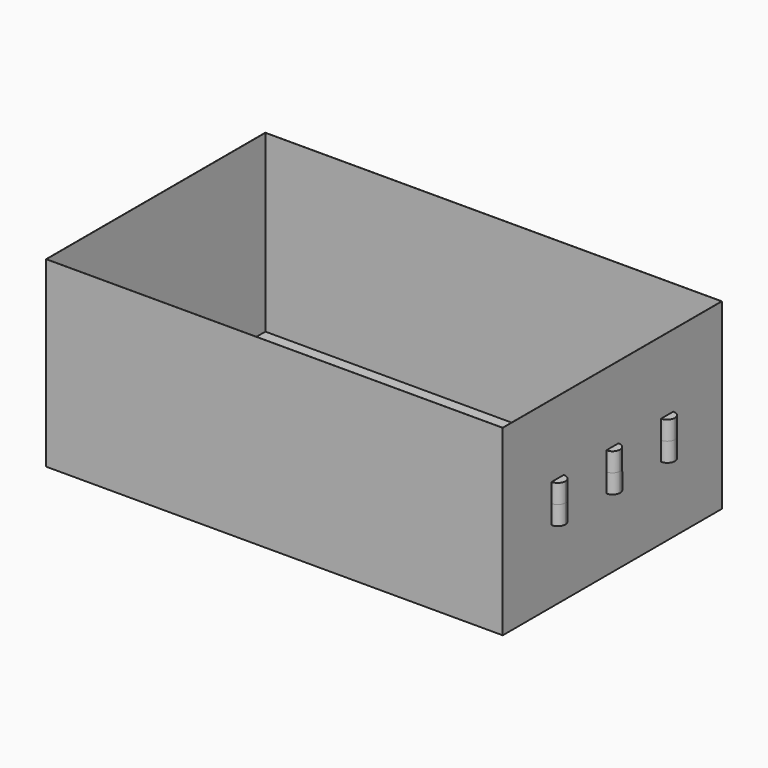
from build123d import *

# Parameters (mm, degrees)
F1_W     = 1524
F1_H     = 914.4
F1_W_2   = 1522.73
F1_H_2   = 913.638
F2_DEPTH = 609.6
F0_W     = 1524
F0_H     = 914.4
F3_DEPTH = 25.4
F6_DEPTH = 63.5


with BuildPart() as f2:
    # F1 (on face) → F2 (new body)
    with BuildSketch(Plane.XY):
        with Locations((694.4408099055, 385.5257871866)):
            Rectangle(F1_W, F1_H)
        with Locations((694.4408099055, 385.5257871866)):
            Rectangle(F1_W_2, F1_H_2, mode=Mode.SUBTRACT)
    extrude(amount=F2_DEPTH)

    # F1 (on face) + F0 (on Top) → F3 (join)
    with BuildSketch(Plane.XY):
        with Locations((694.4408099055, 385.5257871866)):
            Rectangle(F1_W_2, F1_H_2)
    with BuildSketch(Plane.XY):
        with Locations((694.4408099055, 385.5257871866)):
            Rectangle(F0_W, F0_H)
    extrude(amount=F3_DEPTH)

    # F5 (on mid) → F6 (join, symmetric)
    with BuildSketch(Plane(origin=(-0.3153710141, -0.1892226085, 302.7561735554), x_dir=(0.9999994575, -6.51e-07, 0.0010416657), z_dir=(0.0010416659, 0.0006249995, -0.9999992622))):
        with BuildLine():
            ThreePointArc((1482.474916731, -157.6878010367), (1475.0354348197, -139.727294641), (1457.0749332675, -132.2878010367))
            Line((1457.0749332675, -132.2878010367), (1457.074916731, -157.6878010367))
            Line((1457.074916731, -157.6878010367), (1457.0749001946, -183.0878010367))
            ThreePointArc((1457.0749001946, -183.0878010367), (1475.0354231266, -175.6483191253), (1482.474916731, -157.6878010367))
        make_face()
        with BuildLine():
            ThreePointArc((1482.4747680271, -386.097211777), (1475.0352861157, -368.1367053814), (1457.0747845635, -360.697211777))
            Line((1457.0747845635, -360.697211777), (1457.0747680271, -386.097211777))
            Line((1457.0747680271, -386.097211777), (1457.0747514906, -411.497211777))
            ThreePointArc((1457.0747514906, -411.497211777), (1475.0352744227, -404.0577298657), (1482.4747680271, -386.097211777))
        make_face()
        with BuildLine():
            ThreePointArc((1482.4746193231, -614.5066225174), (1475.0351374118, -596.5461161218), (1457.0746358596, -589.1066225174))
            Line((1457.0746358596, -589.1066225174), (1457.0746193231, -614.5066225174))
            Line((1457.0746193231, -614.5066225174), (1457.0746027867, -639.9066225174))
            ThreePointArc((1457.0746027867, -639.9066225174), (1475.0351257188, -632.467140606), (1482.4746193231, -614.5066225174))
        make_face()
        with BuildLine():
            Line((1457.0746193231, -614.5066225174), (1457.0746358596, -589.1066225174))
            ThreePointArc((1457.0746358596, -589.1066225174), (1431.6746193231, -614.5066059809), (1457.0746027867, -639.9066225174))
            Line((1457.0746027867, -639.9066225174), (1457.0746193231, -614.5066225174))
        make_face()
        with BuildLine():
            Line((1457.0747680271, -386.097211777), (1457.0747845635, -360.697211777))
            ThreePointArc((1457.0747845635, -360.697211777), (1431.6747680271, -386.0971952406), (1457.0747514906, -411.497211777))
            Line((1457.0747514906, -411.497211777), (1457.0747680271, -386.097211777))
        make_face()
        with BuildLine():
            Line((1457.074916731, -157.6878010367), (1457.0749332675, -132.2878010367))
            ThreePointArc((1457.0749332675, -132.2878010367), (1431.674916731, -157.6877845002), (1457.0749001946, -183.0878010367))
            Line((1457.0749001946, -183.0878010367), (1457.074916731, -157.6878010367))
        make_face()
    extrude(amount=F6_DEPTH, both=True)


solid = f2.part
